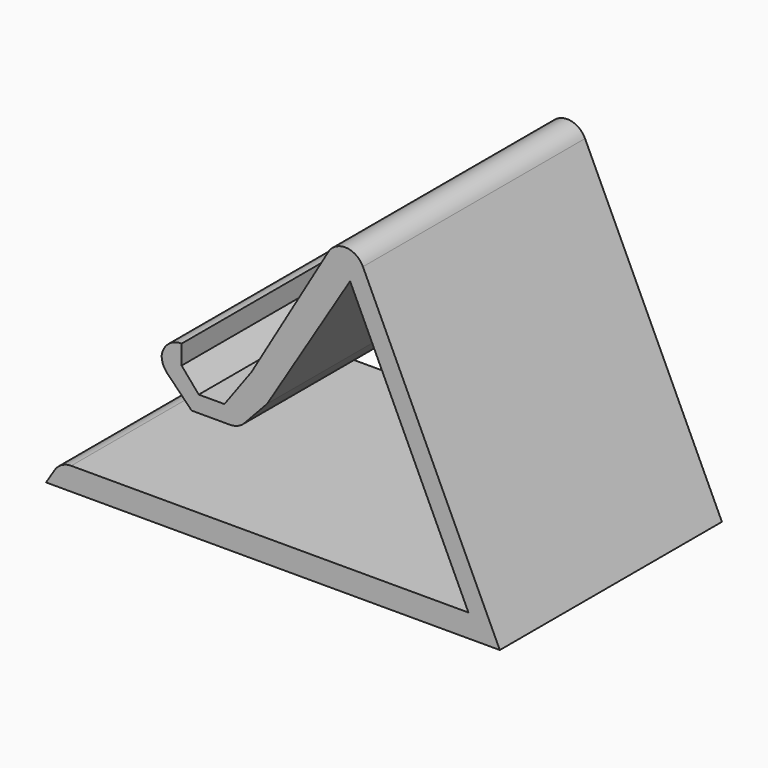
from build123d import *

# Parameters (mm, degrees)
F1_DEPTH    = 71.882
F2_R        = 5.08
F3_T1_DEPTH = 112.7375789557
F3_T3_DEPTH = 85.95990044
F3_T5_DEPTH = 120.1718750332
F3_T7_DEPTH = 82.9446926806


# Not quite as in the source:
# - a fillet or chamfer that OpenCascade refuses, or shapes differently, is made with other operations: its cross-section is extruded or revolved along the edge and cut away or added


with BuildPart() as f1:
    # F0 (on Front) → F1 (new body)
    with BuildSketch(Plane.XZ):
        Polygon((-35.8331985772, 9.4200642779), (-35.8331985772, 14.96128086), (-41.0050004721, 17.5471808761), (-41.0050004721, 7.9424064606), (-33.2472957671, 0), (-21.0566222668, 0), (-13.6683331802, 7.9424064606), (7.7815425405, 42.8511098702), (38.4191013873, -22.7189920843), (-67.233428359, -22.7189920843), (-70.92756778, -28.6296233535), (46.5462207794, -28.6296233535), (7.0188767277, 55.9662804008), (-17.7318900824, 13.8530377299), (-24.750765413, 4.2482619174), (-31.4002260566, 4.2482619174), align=None)
    extrude(amount=F1_DEPTH)

    # F2
    f2_edges = [f1.edges().sort_by_distance(p)[0] for p in [
        (-41.005, -35.941, 7.942406),
    ]]
    fillet(f2_edges, radius=F2_R)

    # F3: fillet of radius 5.08 on 4 edges, made by hand

    # F3_s2 → F3_t1 (cut)
    with BuildSketch(Plane.XZ.offset(-20.4277894779)):
        with BuildLine():
            ThreePointArc((-41.0050004721, 10.0116893284), (-38.3510310012, 13.8358325022), (-33.6965318012, 13.8929478568))
            Line((-33.6965318012, 13.8929478568), (-41.0050004721, 17.5471808761))
            Line((-41.0050004721, 17.5471808761), (-41.0050004721, 10.0116893284))
        make_face()
    extrude(amount=F3_T1_DEPTH, mode=Mode.SUBTRACT)

    # F3_s4 → F3_t3 (cut)
    with BuildSketch(Plane.XZ.offset(-7.03895022)):
        with BuildLine():
            ThreePointArc((-64.417848271, -22.7189920843), (-66.8804738001, -23.3558090469), (-68.7256813332, -25.1066001536))
            Line((-68.7256813332, -25.1066001536), (-67.233428359, -22.7189920843))
            Line((-67.233428359, -22.7189920843), (-64.417848271, -22.7189920843))
        make_face()
    extrude(amount=F3_T3_DEPTH, mode=Mode.SUBTRACT)

    # F3_s6 → F3_t5 (cut)
    with BuildSketch(Plane.XZ.offset(-24.1449375166)):
        with BuildLine():
            ThreePointArc((2.1252810988, 47.6398644221), (6.7441636939, 50.1402432188), (11.1072770532, 47.2163396005))
            Line((11.1072770532, 47.2163396005), (7.0188767277, 55.9662804008))
            Line((7.0188767277, 55.9662804008), (2.1252810988, 47.6398644221))
        make_face()
    extrude(amount=F3_T5_DEPTH, mode=Mode.SUBTRACT)

    # F3_s8 → F3_t7 (cut)
    with BuildSketch(Plane.XZ.offset(-5.5313463403)):
        with BuildLine():
            ThreePointArc((-23.2691608029, 0), (-21.2406694782, 0.4225733558), (-19.5496531088, 1.6199909663))
            Line((-19.5496531088, 1.6199909663), (-21.0566222668, 0))
            Line((-21.0566222668, 0), (-23.2691608029, 0))
        make_face()
    extrude(amount=F3_T7_DEPTH, mode=Mode.SUBTRACT)


solid = f1.part
